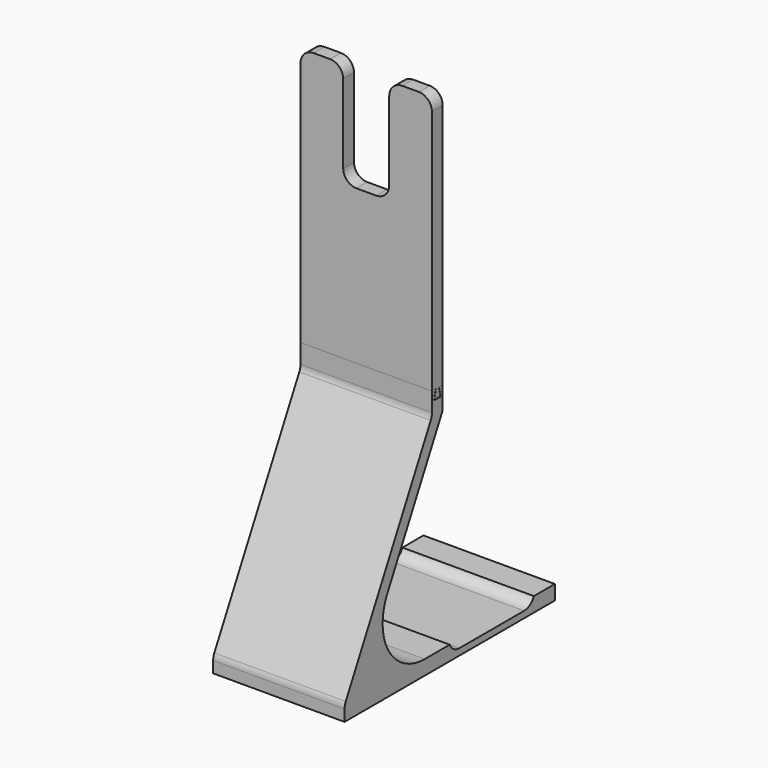
from build123d import *

# Parameters (mm, degrees)
F1_DEPTH    = 100
F2_T1_DEPTH = 100
F2_T3_DEPTH = 100
F2_T5_DEPTH = 100
F2_T7_DEPTH = 112.2298810339
F2_T9_DEPTH = 112.2298810339
F4_DEPTH    = 100
F5_W        = 35
F5_H        = 80
F6_DEPTH    = 25
F7_R        = 10
F8_R        = 40


# Not quite as in the source:
# - a fillet or chamfer that OpenCascade refuses, or shapes differently, is made with other operations: its cross-section is extruded or revolved along the edge and cut away or added


with BuildPart() as f1:
    # F0 (on Right) → F1 (new body)
    with BuildSketch(Plane.YZ):
        Polygon((136.5221505807, -29.5914116513), (136.5221505807, -18.4788270524), (116.5221505807, -18.4788270524), (116.5221505807, -24.5914116513), (36.5221505807, -24.5914116513), (36.5221505807, -18.4788270524), (-53.1987108176, -18.4788270524), (-63.4778494193, -18.4788270524), (-63.4778494193, -29.5914116513), align=None)
        Polygon((19.6065225478, 158.2476049662), (19.6065225478, 141.1989332489), (29.8856611494, 141.1989332489), (29.8856611494, 158.2476049662), (26.3856611494, 158.2476049662), (27.8856611494, 151.2272953987), (21.6065225478, 151.2272953987), (23.1065225478, 158.2476049662), align=None)
        Polygon((19.6065225478, 141.1989332489), (-63.4778494193, -18.4788270524), (-53.1987108176, -18.4788270524), (29.8856611494, 141.1989332489), align=None)
    extrude(amount=F1_DEPTH)

    # F2: fillet of radius 10 on 5 edges, made by hand

    # F2_s2 → F2_t1 (join)
    with BuildSketch(Plane.YZ):
        with BuildLine():
            ThreePointArc((116.5221505807, -18.4788270524), (112.8370564508, -22.9243029266), (107.3086820971, -24.5914116513))
            Line((107.3086820971, -24.5914116513), (116.5221505807, -24.5914116513))
            Line((116.5221505807, -24.5914116513), (116.5221505807, -18.4788270524))
        make_face()
    extrude(amount=F2_T1_DEPTH)

    # F2_s4 → F2_t3 (join)
    with BuildSketch(Plane.YZ):
        with BuildLine():
            ThreePointArc((45.7356190644, -24.5914116513), (40.2072447107, -22.9243029266), (36.5221505807, -18.4788270524))
            Line((36.5221505807, -18.4788270524), (36.5221505807, -24.5914116513))
            Line((36.5221505807, -24.5914116513), (45.7356190644, -24.5914116513))
        make_face()
    extrude(amount=F2_T3_DEPTH)

    # F2_s6 → F2_t5 (join)
    with BuildSketch(Plane.YZ):
        with BuildLine():
            ThreePointArc((19.6065225478, 143.6449094556), (19.3201693098, 141.2689745696), (18.4775092312, 139.029111013))
            Line((18.4775092312, 139.029111013), (19.6065225478, 141.1989332489))
            Line((19.6065225478, 141.1989332489), (19.6065225478, 143.6449094556))
        make_face()
    extrude(amount=F2_T5_DEPTH)

    # F2_s8 → F2_t7 (cut)
    with BuildSketch(Plane.YZ.offset(-6.114940517)):
        with BuildLine():
            ThreePointArc((28.7566478328, 139.029111013), (29.5993079114, 141.2689745696), (29.8856611494, 143.6449094556))
            Line((29.8856611494, 143.6449094556), (29.8856611494, 141.1989332489))
            Line((29.8856611494, 141.1989332489), (28.7566478328, 139.029111013))
        make_face()
    extrude(amount=F2_T7_DEPTH, mode=Mode.SUBTRACT)

    # F2_s10 → F2_t9 (cut)
    with BuildSketch(Plane.YZ.offset(-6.114940517)):
        with BuildLine():
            ThreePointArc((-63.4778494193, -20.9248032592), (-63.1914961813, -18.5488683731), (-62.3488361027, -16.3090048166))
            Line((-62.3488361027, -16.3090048166), (-63.4778494193, -18.4788270524))
            Line((-63.4778494193, -18.4788270524), (-63.4778494193, -20.9248032592))
        make_face()
    extrude(amount=F2_T9_DEPTH, mode=Mode.SUBTRACT)

    # F8
    f8_edges = [f1.edges().sort_by_distance(p)[0] for p in [
        (50, -53.198711, -18.478827),
    ]]
    fillet(f8_edges, radius=F8_R)


with BuildPart() as f4:
    # F3 (on face) → F4 (new body)
    with BuildSketch(Plane.YZ):
        Polygon((29.8856611494, 355.4085883487), (19.6065225478, 355.4085883487), (19.6065225478, 158.2476049662), (23.1065225478, 158.2476049662), (23.3065225478, 158.2476049662), (21.8278891269, 151.4272953987), (24.5640873909, 151.4272953987), (27.6642945703, 151.4272953987), (26.1856611494, 158.2476049662), (26.3856611494, 158.2476049662), (29.8856611494, 158.2476049662), align=None)
    extrude(amount=F4_DEPTH)

    # F5 (on face) → F6 (cut)
    with BuildSketch(Plane(origin=(0, 29.8856611494, 0), x_dir=(-1, 0, 0), z_dir=(0, 1, 0))):
        with Locations((-50, 315.4085883487)):
            Rectangle(F5_W, F5_H)
    extrude(amount=-F6_DEPTH, mode=Mode.SUBTRACT)

    # F7
    f7_edges = [f4.edges().sort_by_distance(p)[0] for p in [
        (32.5, 24.746092, 275.408588),
        (67.5, 24.746092, 275.408588),
        (32.5, 24.746092, 355.408588),
        (67.5, 24.746092, 355.408588),
        (100, 24.746092, 355.408588),
        (0, 24.746092, 355.408588),
    ]]
    fillet(f7_edges, radius=F7_R)


solid = Compound([f1.part, f4.part])
